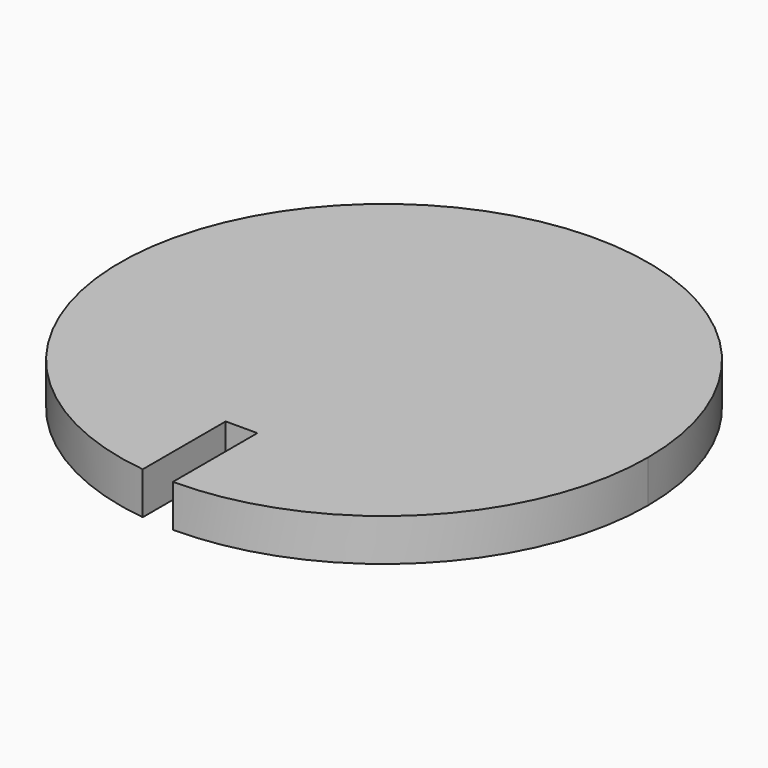
from build123d import *

# Parameters (mm, degrees)
F0_R     = 25
F1_DEPTH = 4
F3_DEPTH = 73


# Not quite as in the source:
# - an extrude ends at something that could not be found from the text; its depth is read off the source's solid


with BuildPart() as f1:
    # F0 (on Top) → F1 (new body)
    with BuildSketch(Plane.XY):
        Circle(F0_R)
    extrude(amount=F1_DEPTH)

    # F2 (on face) → F3 (cut, through all)
    with BuildSketch(Plane.XY.offset(4)):
        with BuildLine():
            Line((-3, -25), (0, -25))
            ThreePointArc((0, -25), (-1.5027171558, -24.9547959549), (-3, -24.819347292))
            Line((-3, -24.819347292), (-3, -25))
        make_face()
        with BuildLine():
            Line((0, -25), (0, -15))
            Line((0, -15), (-3, -15))
            Line((-3, -15), (-3, -24.819347292))
            ThreePointArc((-3, -24.819347292), (-1.5027171558, -24.9547959549), (0, -25))
        make_face()
    extrude(amount=-F3_DEPTH, mode=Mode.SUBTRACT)


solid = f1.part
